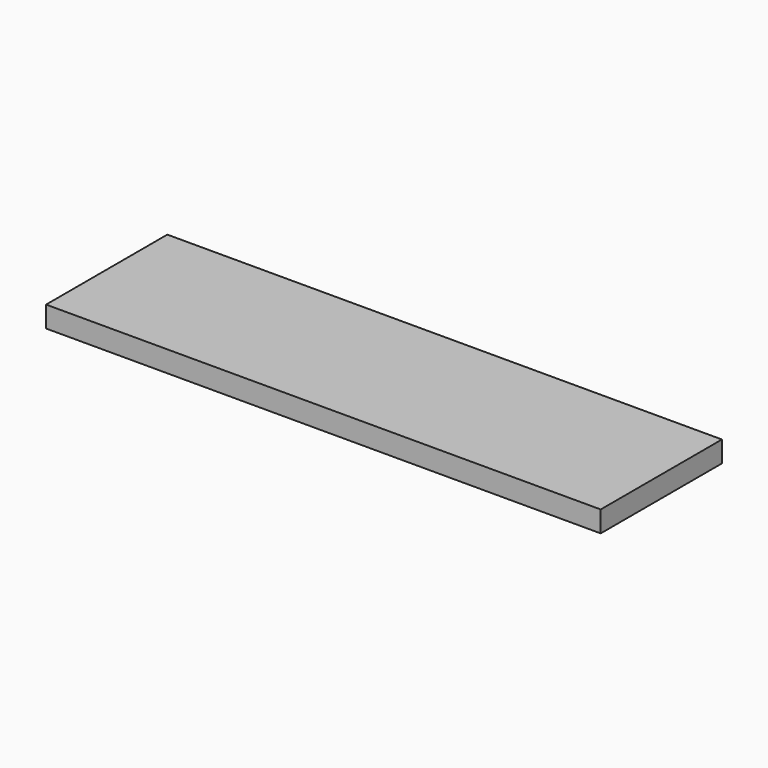
from build123d import *

# Parameters (mm, degrees)
F0_W         = 120.2385276556
F0_H         = 32.8527437523
F1_DEPTH     = 4.572
F2_TEXT_SIZE = 26.0904120902
F3_DEPTH     = 2.286


# Not quite as in the source:
# - Text() gives the source's letters only with a copy of the font that has no kerning and outlines rounded to 1/6400 em; it was checked with that copy


with BuildPart() as f1:
    # F0 (on Top) → F1 (new body)
    with BuildSketch(Plane.XY):
        with Locations((9.3128085136, -22.2832537256)):
            Rectangle(F0_W, F0_H)
    extrude(amount=-F1_DEPTH)

    # F2 (on face) → F3 (join)
    with BuildSketch(Plane(origin=(0, 0, -4.572), x_dir=(1, 0, 0), z_dir=(0, 0, -1))):
        with Locations((-37.295669812, 14.4684594125)):
            Text('Jorge O', F2_TEXT_SIZE, font='Open Sans', text_align=(TextAlign.LEFT, TextAlign.BOTTOM))
    extrude(amount=F3_DEPTH)


solid = f1.part
